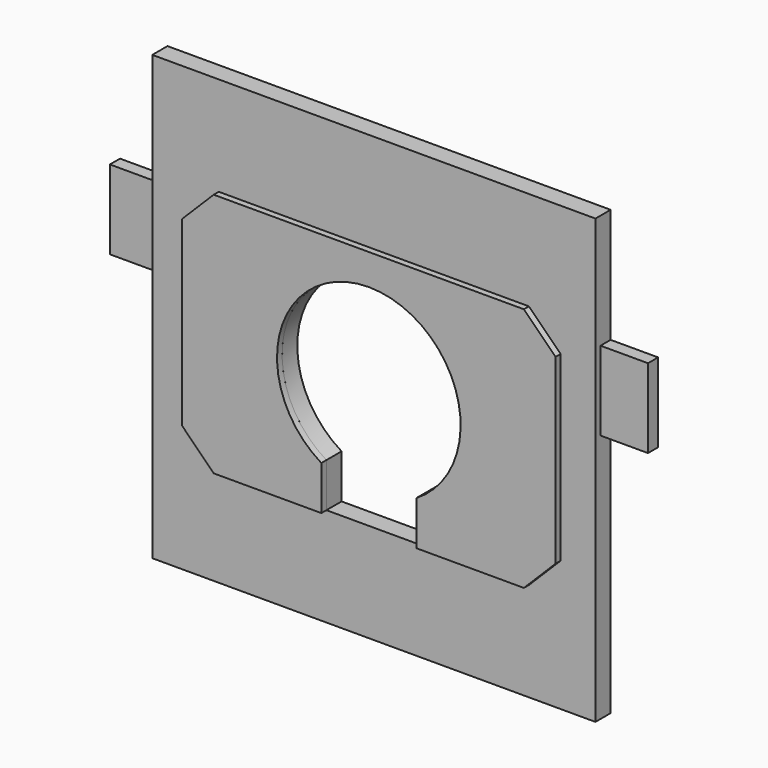
from build123d import *

# Parameters (mm, degrees)
F0_W     = 280
F0_H     = 280
F1_DEPTH = 12
F2_W     = 236
F2_H     = 155
F2_R     = 58
F3_DEPTH = 4
F4_SIZE  = 20
F5_W     = 30
F5_H     = 50
F6_DEPTH = 8
F8_DEPTH = 16.001
F9_DEPTH = 449


# Not quite as in the source:
# - an extrude ends at something that could not be found from the text; its depth is read off the source's solid


with BuildPart() as f1:
    # F0 (on Front) → F1 (new body)
    with BuildSketch(Plane.XZ):
        Rectangle(F0_W, F0_H)
        with BuildLine():
            ThreePointArc((-30, -49.638694584), (-28.4956136976, 50.5173237613), (58, 0))
            ThreePointArc((58, 0), (50.5173237613, -28.4956136976), (30, -49.638694584))
            Line((30, -49.638694584), (30, -77.5))
            Line((30, -77.5), (-30, -77.5))
            Line((-30, -77.5), (-30, -49.638694584))
        make_face(mode=Mode.SUBTRACT)
    extrude(amount=F1_DEPTH)

    # F5 (on face) → F6 (join)
    with BuildSketch(Plane(origin=(0, 0, 0), x_dir=(-1, 0, 0), z_dir=(0, 1, 0))):
        with Locations((-155, 42.6539830863)):
            Rectangle(F5_W, F5_H)
        with Locations((155, 42.6539830863)):
            Rectangle(F5_W, F5_H)
    extrude(amount=-F6_DEPTH)

    # F0 (on Front) → F9 (cut, through all)
    with BuildSketch(Plane.XZ):
        with BuildLine():
            ThreePointArc((30, -49.638694584), (0, -58), (-30, -49.638694584))
            Line((-30, -49.638694584), (-30, -77.5))
            Line((-30, -77.5), (30, -77.5))
            Line((30, -77.5), (30, -49.638694584))
        make_face()
    extrude(amount=-F9_DEPTH, mode=Mode.SUBTRACT)


with BuildPart() as f3:
    # F2 (on face) → F3 (new body)
    with BuildSketch(Plane.XZ.offset(12)):
        Rectangle(F2_W, F2_H)
        Circle(F2_R, mode=Mode.SUBTRACT)
    extrude(amount=F3_DEPTH)

    # F4
    f4_edges = [f3.edges().sort_by_distance(p)[0] for p in [
        (118, -14, -77.5),
        (-118, -14, -77.5),
        (118, -14, 77.5),
        (-118, -14, 77.5),
    ]]
    chamfer(f4_edges, length=F4_SIZE)

    # F7 (on face) → F8 (cut, through all)
    with BuildSketch(Plane.XZ.offset(16)):
        with BuildLine():
            ThreePointArc((30, -49.638694584), (0, -58), (-30, -49.638694584))
            Line((-30, -49.638694584), (-30, -77.5))
            Line((-30, -77.5), (30, -77.5))
            Line((30, -77.5), (30, -49.638694584))
        make_face()
    extrude(amount=-F8_DEPTH, mode=Mode.SUBTRACT)


solid = Compound([f1.part, f3.part])
